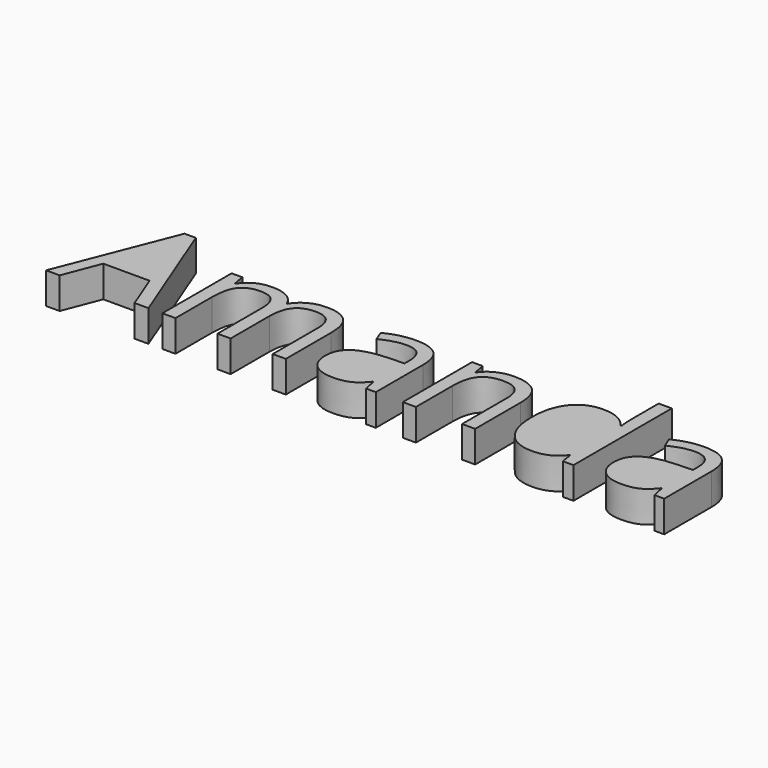
from build123d import *

# Parameters (mm, degrees)
F0_TEXT_SIZE = 25.7358854753
F1_DEPTH     = 5


# Not quite as in the source:
# - Text() gives the source's letters only with a copy of the font that has no kerning and outlines rounded to 1/6400 em; it was checked with that copy


with BuildPart() as f1:
    # F0 (on Top) → F1 (new body)
    with BuildSketch(Plane.XY):
        with BuildLine():
            add(Edge.make_bspline(
                [(25.0387949126, -5.5589970449), (26.005901234, -6.9040991841), (27.8797953952, -6.9040991841)],
                knots=[0, 0, 0, 1, 1, 1], degree=2))
            add(Edge.make_bspline(
                [(27.8797953952, -6.9040991841), (30.0150696432, -6.9040991841), (30.9761441164, -5.7419631057)],
                knots=[0, 0, 0, 1, 1, 1], degree=2))
            add(Edge.make_bspline(
                [(30.9761441164, -5.7419631057), (31.9372185896, -4.5798270272), (31.9372185896, -1.9901535512)],
                knots=[0, 0, 0, 1, 1, 1], degree=2))
            Line((31.9372185896, -1.9901535512), (31.9372185896, -1.5518392517))
            add(Edge.make_bspline(
                [(31.9372185896, -1.5518392517), (31.9372185896, 1.3756177211), (30.9640804201, 2.6262209059)],
                knots=[0, 0, 0, 1, 1, 1], degree=2))
            add(Edge.make_bspline(
                [(30.9640804201, 2.6262209059), (29.9909422506, 3.8768240907), (27.8556680025, 3.8768240907)],
                knots=[0, 0, 0, 1, 1, 1], degree=2))
            add(Edge.make_bspline(
                [(27.8556680025, 3.8768240907), (26.0179649303, 3.8768240907), (25.0448267608, 2.4512973093)],
                knots=[0, 0, 0, 1, 1, 1], degree=2))
            add(Edge.make_bspline(
                [(25.0448267608, 2.4512973093), (24.0716885913, 1.0257705279), (24.0716885913, -1.5759666443)],
                knots=[0, 0, 0, 1, 1, 1], degree=2))
            add(Edge.make_bspline(
                [(24.0716885913, -1.5759666443), (24.0716885913, -4.2138949056), (25.0387949126, -5.5589970449)],
                knots=[0, 0, 0, 1, 1, 1], degree=2))
        make_face()
        with Locations((-49.8667061329, -8.3999975274)):
            Text('Amanda', F0_TEXT_SIZE, font='Open Sans', text_align=(TextAlign.LEFT, TextAlign.BOTTOM))
        with BuildLine():
            add(Edge.make_bspline(
                [(40.2893176728, -6.3391160733), (40.9729271307, -6.9282265768), (42.203424155, -6.9282265768)],
                knots=[0, 0, 0, 1, 1, 1], degree=2))
            add(Edge.make_bspline(
                [(42.203424155, -6.9282265768), (44.1537217262, -6.9282265768), (45.2655924034, -5.8605894528)],
                knots=[0, 0, 0, 1, 1, 1], degree=2))
            add(Edge.make_bspline(
                [(45.2655924034, -5.8605894528), (46.3774630806, -4.7929523288), (46.3774630806, -2.8708033823)],
                knots=[0, 0, 0, 1, 1, 1], degree=2))
            Line((46.3774630806, -2.8708033823), (46.3774630806, -1.6282426617))
            Line((46.3774630806, -1.6282426617), (44.2904436178, -1.7126885359))
            add(Edge.make_bspline(
                [(44.2904436178, -1.7126885359), (41.8013009445, -1.8011556422), (40.7035045797, -2.4867757162)],
                knots=[0, 0, 0, 1, 1, 1], degree=2))
            add(Edge.make_bspline(
                [(40.7035045797, -2.4867757162), (39.6057082149, -3.1723957902), (39.6057082149, -4.6160181161)],
                knots=[0, 0, 0, 1, 1, 1], degree=2))
            add(Edge.make_bspline(
                [(39.6057082149, -4.6160181161), (39.6057082149, -5.7500055699), (40.2893176728, -6.3391160733)],
                knots=[0, 0, 0, 1, 1, 1], degree=2))
        make_face()
        with BuildLine():
            add(Edge.make_bspline(
                [(-5.588919419, -6.3391160733), (-4.9053099611, -6.9282265768), (-3.6748129368, -6.9282265768)],
                knots=[0, 0, 0, 1, 1, 1], degree=2))
            add(Edge.make_bspline(
                [(-3.6748129368, -6.9282265768), (-1.7245153656, -6.9282265768), (-0.6126446885, -5.8605894528)],
                knots=[0, 0, 0, 1, 1, 1], degree=2))
            add(Edge.make_bspline(
                [(-0.6126446885, -5.8605894528), (0.4992259887, -4.7929523288), (0.4992259887, -2.8708033823)],
                knots=[0, 0, 0, 1, 1, 1], degree=2))
            Line((0.4992259887, -2.8708033823), (0.4992259887, -1.6282426617))
            Line((0.4992259887, -1.6282426617), (-1.5877934741, -1.7126885359))
            add(Edge.make_bspline(
                [(-1.5877934741, -1.7126885359), (-4.0769361474, -1.8011556422), (-5.1747325122, -2.4867757162)],
                knots=[0, 0, 0, 1, 1, 1], degree=2))
            add(Edge.make_bspline(
                [(-5.1747325122, -2.4867757162), (-6.272528877, -3.1723957902), (-6.272528877, -4.6160181161)],
                knots=[0, 0, 0, 1, 1, 1], degree=2))
            add(Edge.make_bspline(
                [(-6.272528877, -4.6160181161), (-6.272528877, -5.7500055699), (-5.588919419, -6.3391160733)],
                knots=[0, 0, 0, 1, 1, 1], degree=2))
        make_face()
        with BuildLine():
            Line((-44.687359181, -0.6349983316), (-38.743978129, -0.6349983316))
            Line((-38.743978129, -0.6349983316), (-40.8832736092, 5.0590663298))
            add(Edge.make_bspline(
                [(-40.8832736092, 5.0590663298), (-41.297460516, 6.1407777661), (-41.7357748155, 7.7090582873)],
                knots=[0, 0, 0, 1, 1, 1], degree=2))
            add(Edge.make_bspline(
                [(-41.7357748155, 7.7090582873), (-42.0132398308, 6.5026886556), (-42.5279575403, 5.0590663298)],
                knots=[0, 0, 0, 1, 1, 1], degree=2))
            Line((-42.5279575403, 5.0590663298), (-44.687359181, -0.6349983316))
        make_face()
    extrude(amount=F1_DEPTH)


solid = f1.part
